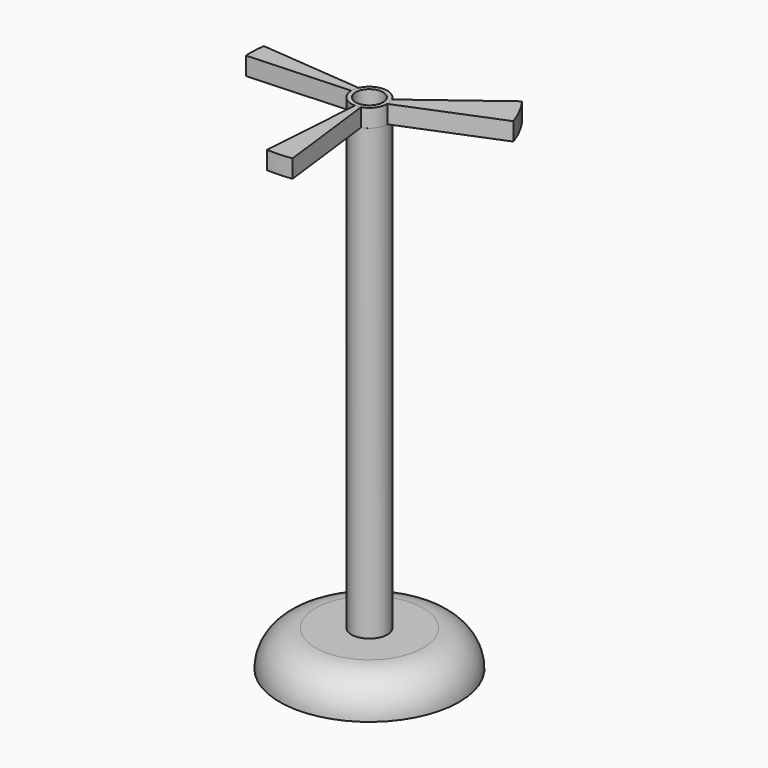
from build123d import *

# Parameters (mm, degrees)
F0_R      = 12.7
F1_DEPTH  = 5.08
F2_R      = 2.54
F3_DEPTH  = 63.5
F4_R      = 1.9341022534
F5_DEPTH  = 66.04
F7_R      = 5.07999
F8_DEPTH  = 2.54
F9_DEPTH  = 2.54
F10_DEPTH = 2.54


# Not quite as in the source:
# - a fillet or chamfer is up to 0.001 mm smaller than in the source, because OpenCascade refuses the exact size
# - the program builds the solid bodies; features that only make, move or delete a surface that nothing else refers to are left out


with BuildPart() as f1:
    # F0 (on Top) → F1 (new body)
    with BuildSketch(Plane.XY):
        Circle(F0_R)
    extrude(amount=F1_DEPTH)

    # F2 (on face) → F3 (join)
    with BuildSketch(Plane.XY.offset(5.08)):
        Circle(F2_R)
    extrude(amount=F3_DEPTH)

    # F4 (on face) → F5 (cut)
    with BuildSketch(Plane.XY.offset(68.58)):
        Circle(F4_R)
    extrude(amount=-F5_DEPTH, mode=Mode.SUBTRACT)

    # F7 (radius 5.08 in the source; OpenCascade refuses exactly that, so slightly less here)
    f7_edges = [f1.edges().sort_by_distance(p)[0] for p in [
        (-12.7, 0, 5.08),
    ]]
    fillet(f7_edges, radius=F7_R)


with BuildPart() as f8:
    # F4 (on face) → F8 (new body)
    with BuildSketch(Plane.XY.offset(68.58)):
        with BuildLine():
            Line((-2.3296703372, 1.0120455128), (-16.7398383993, 2.2762761567))
            ThreePointArc((-16.7398383993, 2.2762761567), (-16.876419297, 0.7681760801), (-16.8774098693, -0.7460957586))
            Line((-16.8774098693, -0.7460957586), (-2.5399770996, -0.0107857982))
            ThreePointArc((-2.5399770996, -0.0107857982), (-2.4879534787, 0.5115539928), (-2.3296703372, 1.0120455128))
        make_face()
    extrude(amount=F8_DEPTH)


with BuildPart() as f9:
    # F4 (on face) → F9 (new body)
    with BuildSketch(Plane.XY.offset(68.58)):
        with BuildLine():
            Line((2.54, 0), (15.9862067387, 5.4630409925))
            ThreePointArc((15.9862067387, 5.4630409925), (15.0355746118, 7.7029292395), (13.7730240822, 9.7830174491))
            Line((13.7730240822, 9.7830174491), (2.2682600086, 1.143064536))
            ThreePointArc((2.2682600086, 1.143064536), (2.4711313625, 0.5874604575), (2.54, 0))
        make_face()
    extrude(amount=F9_DEPTH)


with BuildPart() as f9b:
    # F4 (on face) → F9, piece 2 (new body)
    with BuildSketch(Plane.XY.offset(68.58)):
        with BuildLine():
            ThreePointArc((-0.990063935, -16.8648568385), (0.7598975693, -16.8767940813), (2.5017050348, -16.7076358201))
            Line((2.5017050348, -16.7076358201), (0.750540077, -2.4265798138))
            ThreePointArc((0.750540077, -2.4265798138), (0.3795308109, -2.5114848922), (0, -2.54))
            Line((0, -2.54), (-0.990063935, -16.8648568385))
        make_face()
    extrude(amount=F9_DEPTH)


with BuildPart() as f10:
    # F4 (on face) → F10 (new body)
    with BuildSketch(Plane.XY.offset(68.58)):
        with BuildLine():
            ThreePointArc((0.750540077, -2.4265798138), (2.0442568082, -1.507519188), (2.54, 0))
            ThreePointArc((2.54, 0), (2.4711313625, 0.5874604575), (2.2682600086, 1.143064536))
            ThreePointArc((2.2682600086, 1.143064536), (-0.0723484846, 2.5389694163), (-2.3296703372, 1.0120455128))
            ThreePointArc((-2.3296703372, 1.0120455128), (-2.4879534787, 0.5115539928), (-2.5399770996, -0.0107857982))
            ThreePointArc((-2.5399770996, -0.0107857982), (-1.7922338118, -1.7998605401), (0, -2.54))
            ThreePointArc((0, -2.54), (0.3795308109, -2.5114848922), (0.750540077, -2.4265798138))
        make_face()
        Circle(F4_R, mode=Mode.SUBTRACT)
    extrude(amount=F10_DEPTH)


solid = Compound([f1.part, f8.part, f9.part, f9b.part, f10.part])
